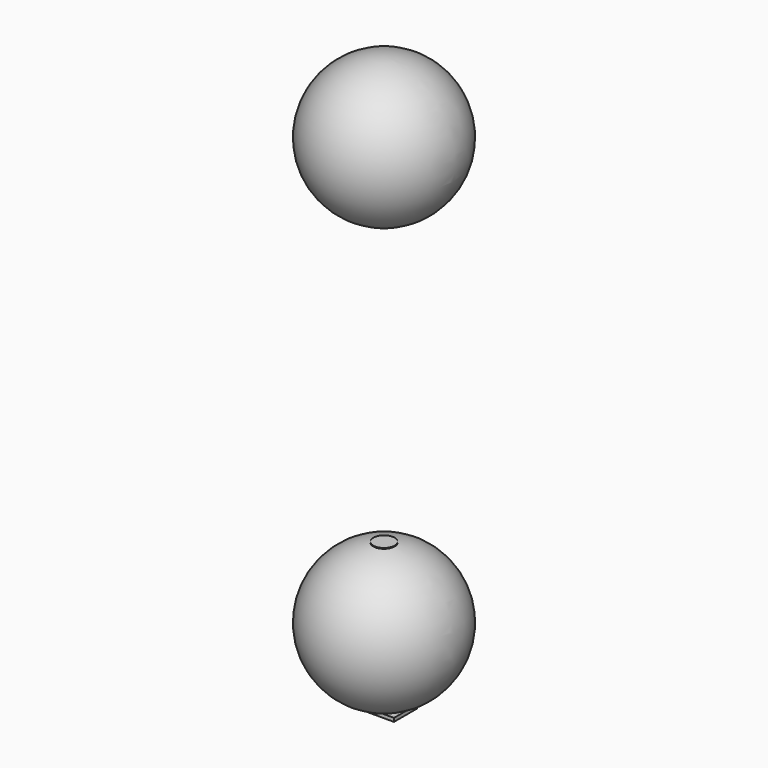
from build123d import *

# Parameters (mm, degrees)
F2_R     = 1.5
F3_DEPTH = 20
F5_W     = 6
F5_H     = 4
F6_DEPTH = 0.5


with BuildPart() as f1:
    # F0 (on Front) → F1 (revolve)
    with BuildSketch(Plane.XZ):
        with BuildLine():
            Line((0, 20), (0, 0))
            ThreePointArc((0, 0), (10, 10), (0, 20))
        make_face()
    revolve(axis=Axis((0, 0, 10), (0, 0, 1)))


with BuildPart() as f1b:
    # F0 (on Front) → F1, piece 2 (revolve)
    with BuildSketch(Plane.XZ):
        with BuildLine():
            Line((0, 80), (0, 60))
            ThreePointArc((0, 60), (10, 70), (0, 80))
        make_face()
    revolve(axis=Axis((0, 0, 10), (0, 0, 1)))


with BuildPart() as f3:
    # F2 (on Top) → F3 (new body)
    with BuildSketch(Plane.XY):
        Circle(F2_R)
    extrude(amount=F3_DEPTH)


with BuildPart() as f1_1:
    add(f1.part)

    # F4: cut F3
    add(f3.part, mode=Mode.SUBTRACT)


with BuildPart() as f3_1:
    add(f3.part)

    # F5 (on Top) → F6 (join)
    with BuildSketch(Plane.XY):
        Rectangle(F5_W, F5_H)
    extrude(amount=-F6_DEPTH)


solid = Compound([f1b.part, f1_1.part, f3_1.part])
